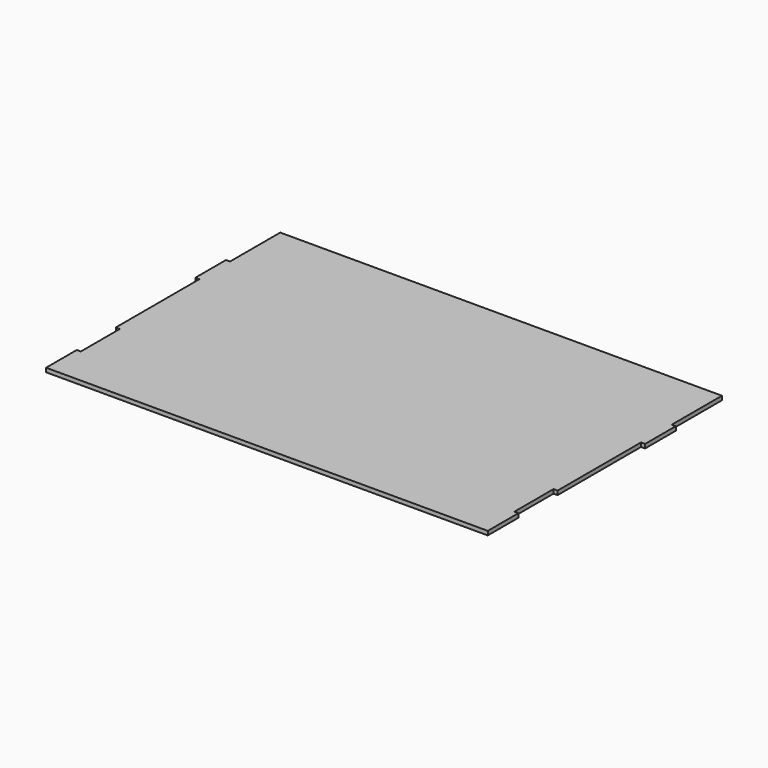
from build123d import *

# Parameters (mm, degrees)
F1_DEPTH = 4.45


# Not quite as in the source:
# - a feature names something its author has since deleted; it is built from what else it names


with BuildPart() as f1:
    # F0 (on Top) → F1 (new body)
    with BuildSketch(Plane.XY):
        Polygon((-238, -73.69707), (238, -73.69707), (242.45, -73.69707), (242.45, -31.63343), (238, -31.63343), (238, -28.2489694095), (238, 22.07074), (242.45, 22.07074), (242.45, 75.69707), (242.45, 77.69707), (242.45, 136.5946788788), (246.9, 136.5946788788), (246.9, 178.6983170484), (242.45, 178.6983170484), (242.45, 237.5959259272), (242.45, 247.5959259272), (232.45, 247.5959259272), (-232.45, 247.5959259272), (-242.45, 247.5959259272), (-242.45, 237.5959259272), (-242.45, 178.6983170484), (-246.9, 178.6983170484), (-246.9, 136.5946788788), (-242.45, 136.5946788788), (-242.45, 75.69707), (-242.45, 22.07074), (-238, 22.07074), (-238, -31.63343), (-242.45, -31.63343), (-242.45, -73.69707), align=None)
    extrude(amount=F1_DEPTH)


solid = f1.part
